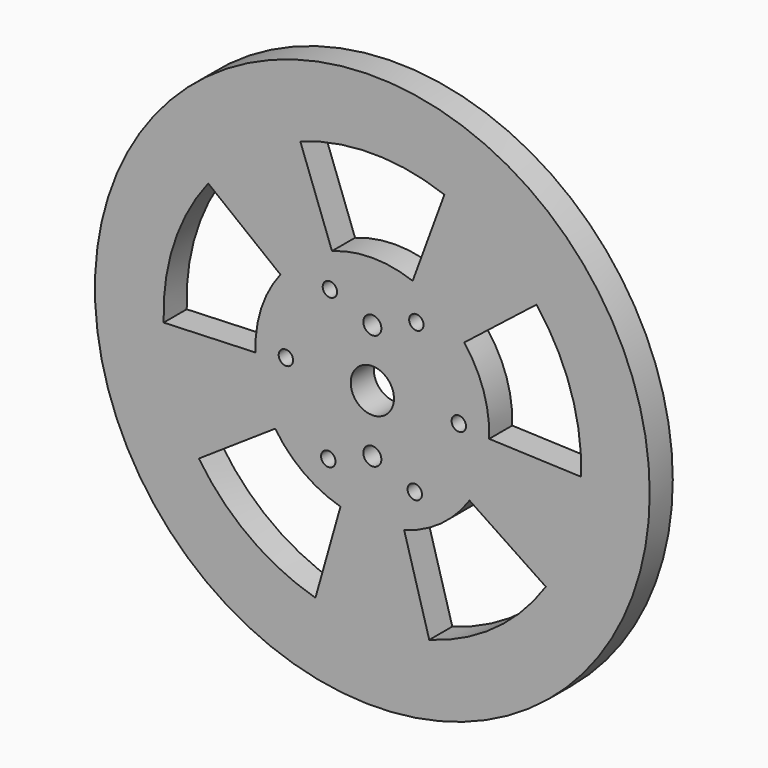
from build123d import *

# Parameters (mm, degrees)
F0_R            = 244.475
F0_R_2          = 6.35
F0_R_3          = 7.9375
F0_R_4          = 19.05
F1_DEPTH        = 25.4
F3_DEPTH        = 25.4
F3_COPIES_COUNT = 5


# Not quite as in the source:
# - a pattern or mirror of a feature is missing from the dataset's text; its kind, count and spacing are read off the source's solid


with BuildPart() as f1:
    # F0 (on Front) → F1 (new body)
    with BuildSketch(Plane.XZ):
        Circle(F0_R)
        with Locations((-38.7905028095, -65.5876275817)):
            Circle(F0_R_2, mode=Mode.SUBTRACT)
        with Locations((37.4053002549, -66.3873746494)):
            Circle(F0_R_2, mode=Mode.SUBTRACT)
        with Locations((0, -50.8)):
            Circle(F0_R_3, mode=Mode.SUBTRACT)
        with Locations((76.1958030644, -0.7997470677)):
            Circle(F0_R_2, mode=Mode.SUBTRACT)
        with Locations((-76.1958030644, 0.7997470677)):
            Circle(F0_R_2, mode=Mode.SUBTRACT)
        with Locations((-37.4053002549, 66.3873746494)):
            Circle(F0_R_2, mode=Mode.SUBTRACT)
        Circle(F0_R_4, mode=Mode.SUBTRACT)
        with Locations((0, 50.8)):
            Circle(F0_R_3, mode=Mode.SUBTRACT)
        with Locations((38.7905028095, 65.5876275817)):
            Circle(F0_R_2, mode=Mode.SUBTRACT)
    extrude(amount=F1_DEPTH)

    # F2 (on Front) → F3 (cut, through all)
    with BuildSketch(Plane.XZ):
        with BuildLine():
            ThreePointArc((-35.5586123208, 96.7233082276), (0, 103.0524782073), (35.5586123208, 96.7233082276))
            Line((35.5586123208, 96.7233082276), (63.5, 172.7269336903))
            ThreePointArc((63.5, 172.7269336903), (0, 184.0294640053), (-63.5, 172.7269336903))
            Line((-63.5, 172.7269336903), (-35.5586123208, 96.7233082276))
        make_face()
    f3 = extrude(amount=F3_DEPTH, mode=Mode.SUBTRACT)

    # F3_copies: F3 ×5 about axis
    f3_copies_axis = Axis((0, 0, 0), (0, 1, 0))
    for i in range(1, F3_COPIES_COUNT):
        add(f3.rotate(f3_copies_axis, i * 360 / F3_COPIES_COUNT), mode=Mode.SUBTRACT)


solid = f1.part
